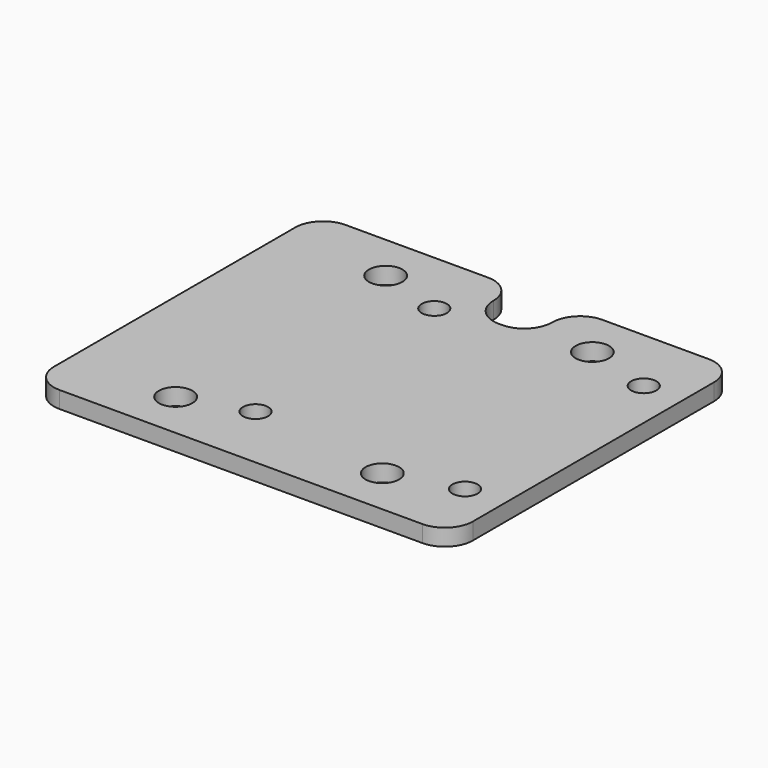
from build123d import *

# Parameters (mm, degrees)
F1_W     = 75
F1_H     = 64
F1_R     = 2.25
F2_DEPTH = 3
F3_R     = 5
F4_R     = 3
F5_DEPTH = 25
F6_W     = 10.5
F6_H     = 12.9868694071
F7_DEPTH = 25
F8_R     = 4.99999


# Not quite as in the source:
# - a fillet or chamfer is up to 0.001 mm smaller than in the source, because OpenCascade refuses the exact size


with BuildPart() as f2:
    # F1 (on Top) → F2 (new body)
    with BuildSketch(Plane.XY):
        with Locations((7, 0)):
            Rectangle(F1_W, F1_H)
        with Locations((0, -20)):
            Circle(F1_R, mode=Mode.SUBTRACT)
        with Locations((37.5, -20)):
            Circle(F1_R, mode=Mode.SUBTRACT)
        with Locations((0, 20)):
            Circle(F1_R, mode=Mode.SUBTRACT)
        with Locations((37.5, 20)):
            Circle(F1_R, mode=Mode.SUBTRACT)
    extrude(amount=F2_DEPTH)

    # F3
    f3_edges = [f2.edges().sort_by_distance(p)[0] for p in [
        (-30.5, 32, 1.5),
        (-30.5, -32, 1.5),
        (44.5, -32, 1.5),
        (44.5, 32, 1.5),
    ]]
    fillet(f3_edges, radius=F3_R)

    # F4 (on Top) → F5 (cut)
    with BuildSketch(Plane.XY):
        with Locations((25.5, 23.5)):
            Circle(F4_R)
        with Locations((-11.5, 23.5)):
            Circle(F4_R)
        with Locations((25.5, -23.5)):
            Circle(F4_R)
        with Locations((-11.5, -23.5)):
            Circle(F4_R)
    extrude(amount=F5_DEPTH, mode=Mode.SUBTRACT)

    # F6 (on Top) → F7 (cut)
    with BuildSketch(Plane.XY):
        with Locations((10.25, 28.4934347035)):
            Rectangle(F6_W, F6_H)
    extrude(amount=F7_DEPTH, mode=Mode.SUBTRACT)

    # F8 (radius 5 in the source; OpenCascade refuses exactly that, so slightly less here)
    f8_edges = [f2.edges().sort_by_distance(p)[0] for p in [
        (5, 32, 1.5),
        (5, 22, 1.5),
        (15.5, 32, 1.5),
        (15.5, 22, 1.5),
    ]]
    fillet(f8_edges, radius=F8_R)


solid = f2.part
